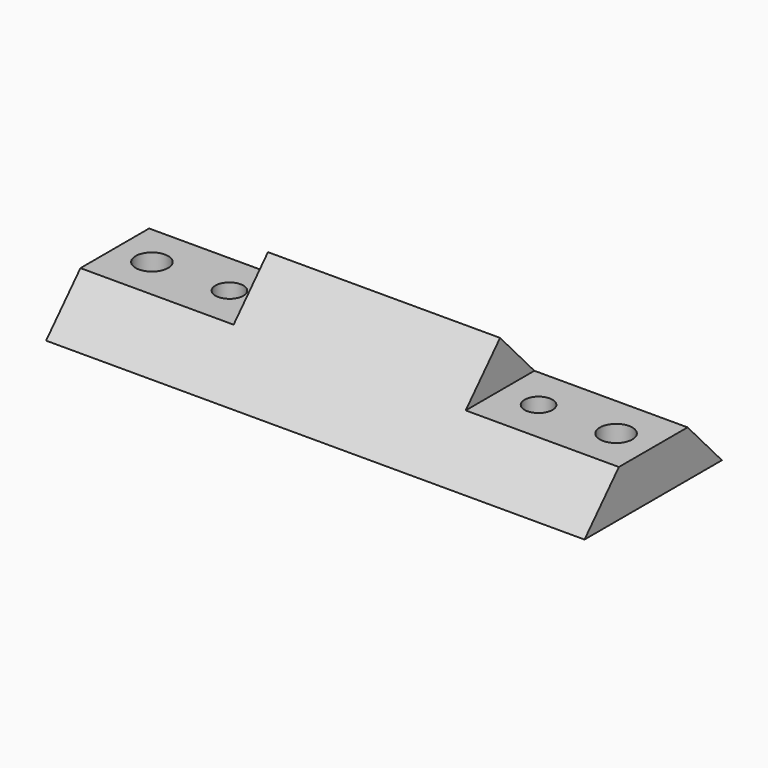
from build123d import *

# Parameters (mm, degrees)
F0_W          = 38
F0_H          = 18.5
F0_R          = 1.5
F0_W_2        = 10
F0_R_2        = 1.75
F1_DEPTH      = 5
F2_W          = 25
F2_H          = 18.5
F3_DEPTH      = 5
F5_DEPTH      = 41.501
F5_DEPTH_BACK = 16.501


with BuildPart() as f1:
    # F0 (on Top) → F1 (new body)
    with BuildSketch(Plane.XY):
        Rectangle(F0_W, F0_H)
        with Locations((-16.65, 0)):
            Circle(F0_R, mode=Mode.SUBTRACT)
        with Locations((16.65, 0)):
            Circle(F0_R, mode=Mode.SUBTRACT)
        with Locations((24, 0)):
            Rectangle(F0_W_2, F0_H)
        with Locations((25, 0)):
            Circle(F0_R_2, mode=Mode.SUBTRACT)
        with Locations((-24, 0)):
            Rectangle(F0_W_2, F0_H)
        with Locations((-25, 0)):
            Circle(F0_R_2, mode=Mode.SUBTRACT)
    extrude(amount=F1_DEPTH)

    # F2 (on face) → F3 (join)
    with BuildSketch(Plane.XY.offset(5)):
        Rectangle(F2_W, F2_H)
    extrude(amount=F3_DEPTH)

    # F4 (on face) → F5 (cut, two sides)
    with BuildSketch(Plane(origin=(-12.5, 0, 0), x_dir=(0, -1, 0), z_dir=(-1, 0, 0))) as f5_sk:
        Polygon((-4.625, 5), (0, 10), (-9.25, 10), (-9.25, 5), align=None)
        Polygon((9.25, 10), (0, 10), (4.625, 5), (9.25, 5), align=None)
        Polygon((9.25, 5), (4.625, 5), (9.25, 0), align=None)
        Polygon((-9.25, 0), (-4.625, 5), (-9.25, 5), align=None)
    extrude(amount=-F5_DEPTH, mode=Mode.SUBTRACT)
    extrude(f5_sk.sketch, amount=F5_DEPTH_BACK, mode=Mode.SUBTRACT)


solid = f1.part
